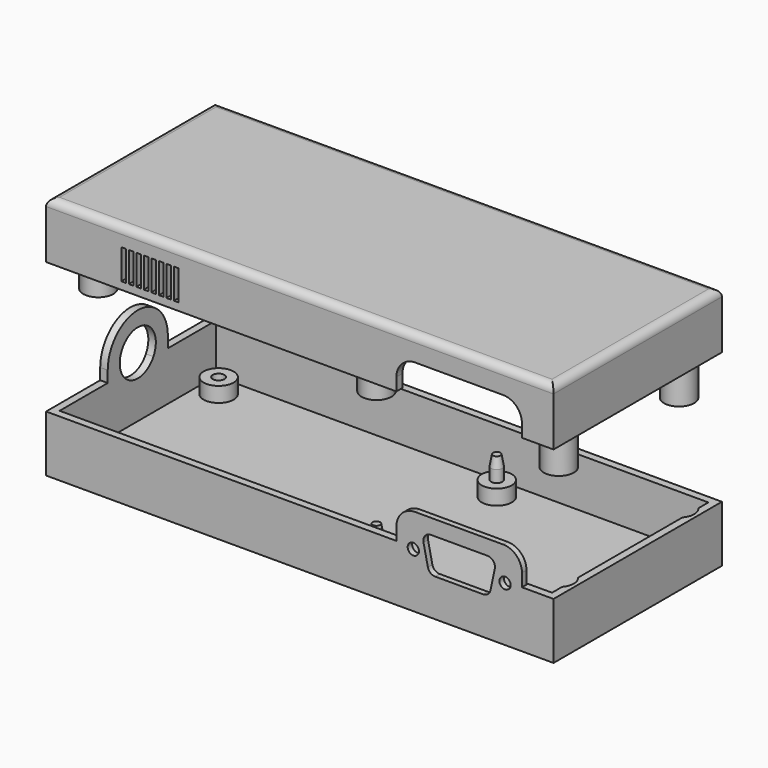
from build123d import *
from build123d import SkipClean  # not in build123d's __all__

# Parameters (mm, degrees)
F0_W        = 135
F0_H        = 56
F1_DEPTH    = 15
F2_T        = -2
F3_R        = 1.5
F4_DEPTH    = 10
F5_R        = 4
F6_DEPTH    = 4
F10_DEPTH   = 5
F8_R        = 1.5
F11_DEPTH   = 1.5
F13_DEPTH   = 25
F15_DEPTH   = 2
F16_W       = 135
F16_H       = 56
F17_DEPTH   = 15
F18_T       = -2
F20_DEPTH   = 5
F22_DEPTH   = 5
F23_R       = 2
F24_R       = 4
F25_DEPTH   = 20
F26_R       = 1.6
F26_R_2     = 1.55
F27_DEPTH   = 15
F28_W       = 1.2
F28_H       = 8
F29_DEPTH   = 100
F31_R       = 4
F32_DEPTH   = 4
F30_R       = 1.55
F33_DEPTH   = 25
F34_R       = 2.85
F35_DEPTH   = 4
F36_R       = 4
F37_DEPTH   = 22
F38_R       = 4
F39_DEPTH   = 25
F40_R       = 1.6
F41_DEPTH   = 22
F43_DEPTH   = 2.6
F44_SIZE2   = 0.5
F44_SIZE    = 2.8356409098
F44_2_SIZE2 = 0.5
F44_2_SIZE  = 2.8356409098


# Not quite as in the source:
# - after a boolean that leaves OpenCascade's solid faulty, fix() repairs it


with BuildPart() as f1:
    # F0 (on Top) → F1 (new body)
    with BuildSketch(Plane.XY):
        with Locations((67.5, 28)):
            Rectangle(F0_W, F0_H)
    extrude(amount=F1_DEPTH)

    # F2
    f2_openings = [f1.faces().sort_by_distance(p)[0] for p in [
        (67.5, 28, 15),
    ]]
    offset(amount=F2_T, openings=f2_openings)

    # F3 (on face) → F4 (join)
    with BuildSketch(Plane.XY.offset(2)):
        with Locations((81.5, 48)):
            Circle(F3_R)
        with Locations((81.5, 8)):
            Circle(F3_R)
        with Locations((7.5, 8)):
            Circle(F3_R)
        with Locations((7.5, 48)):
            Circle(F3_R)
    extrude(amount=F4_DEPTH)

    # F5 (on face) → F6 (join)
    with BuildSketch(Plane.XY.offset(2)):
        with Locations((81.5, 48)):
            Circle(F5_R)
        with Locations((81.5, 8)):
            Circle(F5_R)
        with Locations((7.5, 48)):
            Circle(F5_R)
        with Locations((7.5, 8)):
            Circle(F5_R)
    extrude(amount=F6_DEPTH)

    # F9 (on face) → F10 (cut)
    with BuildSketch(Plane.XZ):
        with BuildLine():
            Line((126.6, 23.4), (93.2, 23.4))
            Line((93.2, 23.4), (93.2, 11))
            ThreePointArc((93.2, 11), (94.6644660941, 7.4644660941), (98.2, 6))
            Line((98.2, 6), (121.6, 6))
            ThreePointArc((121.6, 6), (125.1355339059, 7.4644660941), (126.6, 11))
            Line((126.6, 11), (126.6, 23.4))
        make_face()
    extrude(amount=-F10_DEPTH, mode=Mode.SUBTRACT)

    # F8 (on face) → F11 (join)
    with BuildSketch(Plane.XZ):
        with BuildLine():
            Line((121.6, 23.4), (98.2, 23.4))
            ThreePointArc((98.2, 23.4), (94.6644660941, 21.9355339059), (93.2, 18.4))
            Line((93.2, 18.4), (93.2, 11))
            ThreePointArc((93.2, 11), (94.6644660941, 7.4644660941), (98.2, 6))
            Line((98.2, 6), (121.6, 6))
            ThreePointArc((121.6, 6), (125.1355339059, 7.4644660941), (126.6, 11))
            Line((126.6, 11), (126.6, 18.4))
            ThreePointArc((126.6, 18.4), (125.1355339059, 21.9355339059), (121.6, 23.4))
        make_face()
        with Locations((97.7, 14.5323744416)):
            Circle(F8_R, mode=Mode.SUBTRACT)
        with BuildLine():
            ThreePointArc((100.413788142, 16.9837847111), (100.8155820096, 18.6584850858), (102.37, 19.4))
            Line((102.37, 19.4), (117.4293995654, 19.4))
            ThreePointArc((117.4293995654, 19.4), (118.9838175558, 18.6584850858), (119.3856114233, 16.9837847111))
            Line((119.3856114233, 16.9837847111), (118.2366752531, 11.5837847111))
            ThreePointArc((118.2366752531, 11.5837847111), (117.5389484809, 10.4455820096), (116.2804633952, 10))
            Line((116.2804633952, 10), (103.5189361702, 10))
            ThreePointArc((103.5189361702, 10), (102.2604510845, 10.4455820096), (101.5627243122, 11.5837847111))
            Line((101.5627243122, 11.5837847111), (100.413788142, 16.9837847111))
        make_face(mode=Mode.SUBTRACT)
        with Locations((122.1, 14.5323744416)):
            Circle(F8_R, mode=Mode.SUBTRACT)
    extrude(amount=-F11_DEPTH)

    # F12 (on face) → F13 (cut)
    with BuildSketch(Plane(origin=(0, 0, 0), x_dir=(0, -1, 0), z_dir=(-1, 0, 0))):
        with BuildLine():
            Line((-22.8038475773, 15), (-33.1961524227, 15))
            ThreePointArc((-33.1961524227, 15), (-28, 12), (-22.8038475773, 15))
        make_face()
    extrude(amount=-F13_DEPTH, mode=Mode.SUBTRACT)

    # F14 (on face) → F15 (join)
    with BuildSketch(Plane(origin=(0, 0, 0), x_dir=(0, -1, 0), z_dir=(-1, 0, 0))):
        with BuildLine():
            ThreePointArc((-33.1961524227, 15), (-29.5529142706, 23.7955549577), (-22, 18))
            ThreePointArc((-22, 18), (-22.2044450423, 16.4470857294), (-22.8038475773, 15))
            Line((-22.8038475773, 15), (-18, 15))
            Line((-18, 15), (-18, 18))
            ThreePointArc((-18, 18), (-28, 28), (-38, 18))
            Line((-38, 18), (-38, 15))
            Line((-38, 15), (-33.1961524227, 15))
        make_face()
    with SkipClean():  # cleaning this boolean's faces spoils the solid; the shape is the same uncleaned
        extrude(amount=-F15_DEPTH)

    # F31 (on face) → F32 (join)
    with BuildSketch(Plane.XY.offset(2)):
        with Locations((130, 48)):
            Circle(F31_R)
        with Locations((130, 8)):
            Circle(F31_R)
    extrude(amount=F32_DEPTH)

    add(f1.part.fix(), mode=Mode.REPLACE)

    # F30 (on face) → F33 (cut)
    with BuildSketch(Plane(origin=(0, 0, 0), x_dir=(1, 0, 0), z_dir=(0, 0, -1))):
        with Locations((7.5, -48)):
            Circle(F30_R)
        with Locations((7.5, -8)):
            Circle(F30_R)
        with Locations((130, -48)):
            Circle(F30_R)
        with Locations((130, -8)):
            Circle(F30_R)
    extrude(amount=-F33_DEPTH, mode=Mode.SUBTRACT)

    # F34 (on face) → F35 (cut)
    with BuildSketch(Plane(origin=(0, 0, 0), x_dir=(1, 0, 0), z_dir=(0, 0, -1))):
        with Locations((7.5, -8)):
            Circle(F34_R)
        with Locations((7.5, -48)):
            Circle(F34_R)
        with Locations((130, -8)):
            Circle(F34_R)
        with Locations((130, -48)):
            Circle(F34_R)
    extrude(amount=-F35_DEPTH, mode=Mode.SUBTRACT)

    # F38 (on face) → F39 (cut)
    with BuildSketch(Plane.XY.offset(6)):
        with Locations((130, 48)):
            Circle(F38_R)
        with Locations((130, 8)):
            Circle(F38_R)
    extrude(amount=F39_DEPTH, mode=Mode.SUBTRACT)

    # F44
    f44_edges = [f1.edges().sort_by_distance(p)[0] for p in [
        (80, 8, 12),
    ]]
    f44_side = f1.faces().sort_by_distance((80, 8, 9))[0]
    chamfer(f44_edges, length=F44_SIZE, length2=F44_SIZE2, reference=f44_side)

    # F44#2
    f44_2_edges = [f1.edges().sort_by_distance(p)[0] for p in [
        (80, 48, 12),
    ]]
    f44_2_side = f1.faces().sort_by_distance((80, 48, 9))[0]
    chamfer(f44_2_edges, length=F44_2_SIZE, length2=F44_2_SIZE2, reference=f44_2_side)


with BuildPart() as f17:
    # F16 (on offset) → F17 (new body)
    with BuildSketch(Plane.XY.offset(50)):
        with Locations((67.5, 28)):
            Rectangle(F16_W, F16_H)
    extrude(amount=F17_DEPTH)

    # F18
    f18_openings = [f17.faces().sort_by_distance(p)[0] for p in [
        (67.5, 28, 50),
    ]]
    offset(amount=F18_T, openings=f18_openings)

    # F19 (on face) → F20 (cut)
    with BuildSketch(Plane(origin=(0, 0, 0), x_dir=(0, -1, 0), z_dir=(-1, 0, 0))):
        with BuildLine():
            Line((-18.2, 50), (-18.2, 52.8))
            ThreePointArc((-18.2, 52.8), (-28, 62.6), (-37.8, 52.8))
            Line((-37.8, 52.8), (-37.8, 50))
            Line((-37.8, 50), (-18.2, 50))
        make_face()
    extrude(amount=-F20_DEPTH, mode=Mode.SUBTRACT)

    # F21 (on face) → F22 (cut)
    with BuildSketch(Plane.XZ):
        with BuildLine():
            Line((93.2, 53.4), (93.2, 50))
            Line((93.2, 50), (126.6, 50))
            Line((126.6, 50), (126.6, 53.4))
            ThreePointArc((126.6, 53.4), (125.1355339059, 56.9355339059), (121.6, 58.4))
            Line((121.6, 58.4), (98.2, 58.4))
            ThreePointArc((98.2, 58.4), (94.6644660941, 56.9355339059), (93.2, 53.4))
        make_face()
    extrude(amount=-F22_DEPTH, mode=Mode.SUBTRACT)

    # F23
    f23_edges = [f17.edges().sort_by_distance(p)[0] for p in [
        (67.5, 56, 65),
        (0, 28, 65),
        (67.5, 0, 65),
        (135, 28, 65),
    ]]
    fillet(f23_edges, radius=F23_R)

    # F24 (on face) → F25 (join)
    with BuildSketch(Plane(origin=(0, 0, 63), x_dir=(1, 0, 0), z_dir=(0, 0, -1))):
        with Locations((81.5, -48)):
            Circle(F24_R)
        with Locations((81.5, -8)):
            Circle(F24_R)
        with Locations((7.5, -48)):
            Circle(F24_R)
        with Locations((7.5, -8)):
            Circle(F24_R)
    extrude(amount=F25_DEPTH)

    # F26 (on face) → F27 (cut)
    with BuildSketch(Plane(origin=(0, 0, 43), x_dir=(1, 0, 0), z_dir=(0, 0, -1))):
        with Locations((81.5, -8)):
            Circle(F26_R)
        with Locations((7.5, -8)):
            Circle(F26_R_2)
        with Locations((7.5, -48)):
            Circle(F26_R_2)
        with Locations((81.5, -48)):
            Circle(F26_R)
    extrude(amount=-F27_DEPTH, mode=Mode.SUBTRACT)

    # F28 (on face) → F29 (cut)
    with BuildSketch(Plane(origin=(0, 56, 0), x_dir=(-1, 0, 0), z_dir=(0, 1, 0))):
        with Locations((-20.6, 56)):
            Rectangle(F28_W, F28_H)
        with Locations((-22.6, 56)):
            Rectangle(F28_W, F28_H)
        with Locations((-24.6, 56)):
            Rectangle(F28_W, F28_H)
        with Locations((-26.6, 56)):
            Rectangle(F28_W, F28_H)
        with Locations((-28.6, 56)):
            Rectangle(F28_W, F28_H)
        with Locations((-30.6, 56)):
            Rectangle(F28_W, F28_H)
        with Locations((-32.6, 56)):
            Rectangle(F28_W, F28_H)
        with Locations((-34.6, 56)):
            Rectangle(F28_W, F28_H)
    extrude(amount=-F29_DEPTH, mode=Mode.SUBTRACT)

    # F36 (on face) → F37 (join)
    with BuildSketch(Plane(origin=(0, 0, 63), x_dir=(1, 0, 0), z_dir=(0, 0, -1))):
        with Locations((130, -8)):
            Circle(F36_R)
        with Locations((130, -48)):
            Circle(F36_R)
    extrude(amount=F37_DEPTH)

    # F40 (on face) → F41 (cut)
    with BuildSketch(Plane(origin=(0, 0, 63), x_dir=(1, 0, 0), z_dir=(0, 0, -1))):
        with Locations((130, -8)):
            Circle(F40_R)
        with Locations((130, -48)):
            Circle(F40_R)
    extrude(amount=F41_DEPTH, mode=Mode.SUBTRACT)

    # F42 (on offset) → F43 (cut)
    with BuildSketch(Plane.XY.offset(50)):
        Polygon((9.1454482672, 10.85), (5.8545517328, 10.85), (2.5, 10.85), (2.5, 5.15), (5.8545517328, 5.15), (9.1454482672, 5.15), (10.7908965344, 8), align=None)
        Polygon((9.1454482672, 50.85), (5.8545517328, 50.85), (2.5, 50.85), (2.5, 45.15), (5.8545517328, 45.15), (9.1454482672, 45.15), (10.7908965344, 48), align=None)
        Polygon((131.6454482672, 10.85), (128.3545517328, 10.85), (125, 10.85), (125, 5.15), (128.3545517328, 5.15), (131.6454482672, 5.15), (133.2908965344, 8), align=None)
        Polygon((131.6454482672, 50.85), (128.3545517328, 50.85), (125, 50.85), (125, 45.15), (128.3545517328, 45.15), (131.6454482672, 45.15), (133.2908965344, 48), align=None)
    extrude(amount=-F43_DEPTH, mode=Mode.SUBTRACT)


solid = Compound([f1.part, f17.part])
